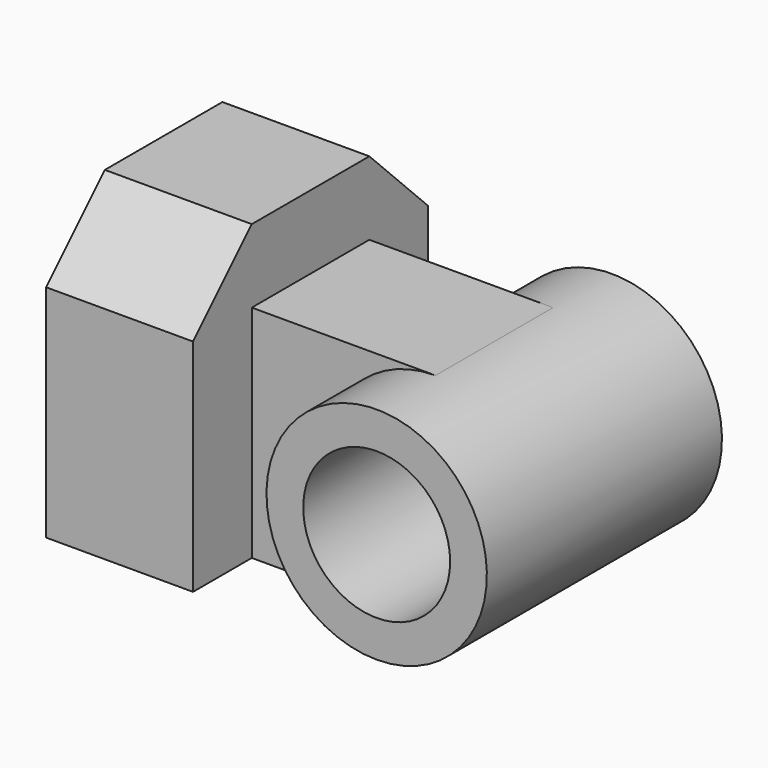
from build123d import *

# Parameters (mm, degrees)
F0_R     = 6.35
F1_DEPTH = 25.4
F3_DEPTH = 6.35
F5_DEPTH = 6.35
F7_DEPTH = 25.4
F9_DEPTH = 25.4


# Not quite as in the source:
# - a pattern or mirror of a feature is missing from the dataset's text; its kind, count and spacing are read off the source's solid
# - a feature names something its author has since deleted; it is built from what else it names


with BuildPart() as f1:
    # F0 (on Front) → F1 (new body)
    with BuildSketch(Plane.XZ):
        Polygon((0, 25.4), (0, 0), (12.7, 0), (12.7, 19.05), (12.7, 25.4), align=None)
        with BuildLine():
            Line((12.7, 19.05), (12.7, 0))
            Line((12.7, 0), (28.575, 0))
            ThreePointArc((28.575, 0), (19.05, 9.525), (28.575, 19.05))
            Line((28.575, 19.05), (12.7, 19.05))
        make_face()
        with BuildLine():
            ThreePointArc((28.575, 19.05), (19.05, 9.525), (28.575, 0))
            ThreePointArc((28.575, 0), (35.3101920908, 2.7898079092), (38.1, 9.525))
            ThreePointArc((38.1, 9.525), (35.3101920908, 16.2601920908), (28.575, 19.05))
        make_face()
        with Locations((28.575, 9.525)):
            Circle(F0_R, mode=Mode.SUBTRACT)
    extrude(amount=F1_DEPTH)

    # F2 (on face) → F3 (cut)
    with BuildSketch(Plane.XZ):
        with BuildLine():
            Line((28.575, 19.05), (12.7, 19.05))
            Line((12.7, 19.05), (12.7, 0))
            Line((12.7, 0), (28.575, 0))
            ThreePointArc((28.575, 0), (19.05, 9.525), (28.575, 19.05))
        make_face()
    extrude(amount=-F3_DEPTH, mode=Mode.SUBTRACT)

    # F4 (on Front) → F5 (cut)
    with BuildSketch(Plane.XZ):
        with BuildLine():
            Line((28.575, 19.05), (12.7, 19.05))
            Line((12.7, 19.05), (12.7, 0))
            Line((12.7, 0), (28.575, 0))
            ThreePointArc((28.575, 0), (19.05, 9.525), (28.575, 19.05))
        make_face()
    f5 = extrude(amount=F5_DEPTH, mode=Mode.SUBTRACT)

    # F5_copies: F5 across plane
    add(f5.mirror(Plane(origin=(0, -12.7, 0), x_dir=(0, 0, -1), z_dir=(0, -1, 0))), mode=Mode.SUBTRACT)

    # F6 (on Right) → F7 (cut)
    with BuildSketch(Plane.YZ):
        Polygon((-25.4, 19.05), (-19.05, 25.4), (-25.4, 25.4), align=None)
    extrude(amount=F7_DEPTH, mode=Mode.SUBTRACT)

    # F8 (on Right) → F9 (cut)
    with BuildSketch(Plane.YZ):
        Polygon((0, 19.05), (0, 25.4), (-6.35, 25.4), align=None)
    extrude(amount=F9_DEPTH, mode=Mode.SUBTRACT)


solid = f1.part
